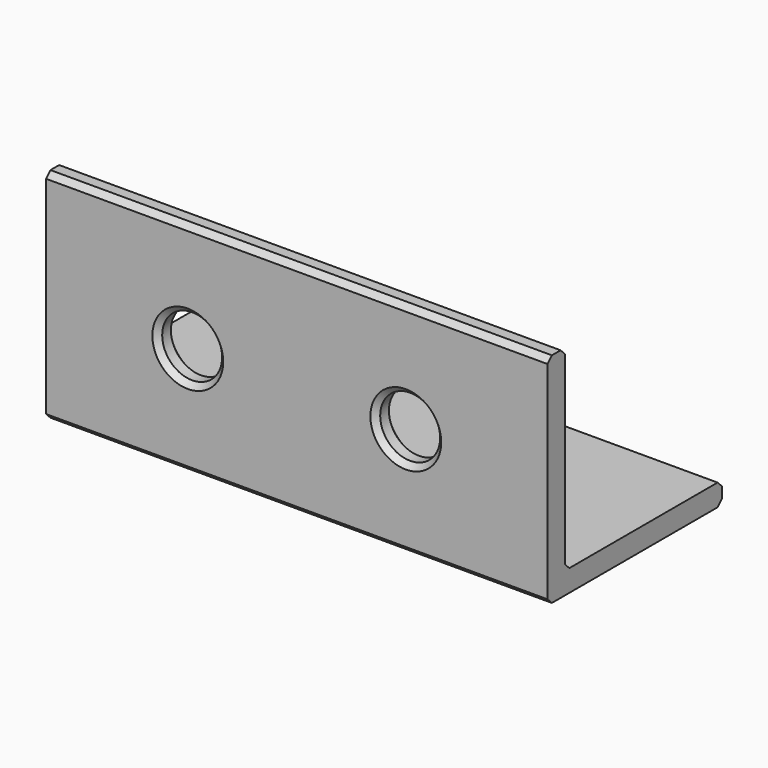
from build123d import *

# Parameters (mm, degrees)
F1_DEPTH  = 50
F2_SIZE   = 0.5
F3_R      = 2.75
F4_DEPTH  = 25
F5_SIZE   = 0.5
F6_R      = 2.75
F7_DEPTH  = 25
F8_SIZE   = 0.5
F9_W      = 1.5
F9_H      = 19
F10_DEPTH = 25


with BuildPart() as f1:
    # F0 (on Right) → F1 (new body)
    with BuildSketch(Plane.YZ):
        Polygon((18, 0), (0, 0), (0, 18), (-2, 18), (-2, -2), (18, -2), align=None)
    extrude(amount=F1_DEPTH)

    # F2
    f2_edges = [f1.edges().sort_by_distance(p)[0] for p in [
        (25, 0, 18),
        (25, -2, 18),
        (0, -1, 18),
        (50, -1, 18),
        (25, 18, 0),
        (25, 0, 0),
        (0, 9, 0),
        (50, 9, 0),
        (25, -2, -2),
        (25, 18, -2),
        (0, 8, -2),
        (50, 8, -2),
        (0, -2, 8),
        (50, -2, 8),
    ]]
    chamfer(f2_edges, length=F2_SIZE)

    # F3 (on face) → F4 (cut)
    with BuildSketch(Plane(origin=(0, 0, 0), x_dir=(-1, 0, 0), z_dir=(0, 1, 0))):
        with Locations((-15, 8)):
            Circle(F3_R)
        with Locations((-35, 8)):
            Circle(F3_R)
    extrude(amount=-F4_DEPTH, mode=Mode.SUBTRACT)

    # F5
    f5_edges = [f1.edges().sort_by_distance(p)[0] for p in [
        (17.75, 0, 8),
        (12.25, -1, 8),
        (17.75, -2, 8),
        (37.75, 0, 8),
        (32.25, -1, 8),
        (37.75, -2, 8),
    ]]
    chamfer(f5_edges, length=F5_SIZE)

    # F6 (on face) → F7 (cut)
    with BuildSketch(Plane(origin=(0, 0, -2), x_dir=(1, 0, 0), z_dir=(0, 0, -1))):
        with Locations((15, -8)):
            Circle(F6_R)
        with Locations((35, -8)):
            Circle(F6_R)
    extrude(amount=-F7_DEPTH, mode=Mode.SUBTRACT)

    # F8
    f8_edges = [f1.edges().sort_by_distance(p)[0] for p in [
        (12.25, 8, -2),
        (17.75, 8, -1),
        (12.25, 8, 0),
        (32.25, 8, -2),
        (37.75, 8, -1),
        (32.25, 8, 0),
    ]]
    chamfer(f8_edges, length=F8_SIZE)

    # F9 (on face) → F10 (cut)
    with BuildSketch(Plane.XZ.offset(2)):
        Polygon((51.7472885549, 18), (48, 18), (48, 17.5), (49.5, 17.5), (49.5, -1.5), (48, -1.5), (48, -2), (48, -2.0400607027), (51.7472885549, -2.0400607027), align=None)
        with Locations((48.75, 8)):
            Rectangle(F9_W, F9_H)
        Polygon((2, 17.5), (2, 18), (2, 19.6672808379), (-2.285732422, 19.6672808379), (-2.285732422, -2), (2, -2), (2, -1.5), (0.5, -1.5), (0.5, 17.5), align=None)
        with Locations((1.25, 8)):
            Rectangle(F9_W, F9_H)
    extrude(amount=-F10_DEPTH, mode=Mode.SUBTRACT)


solid = f1.part
